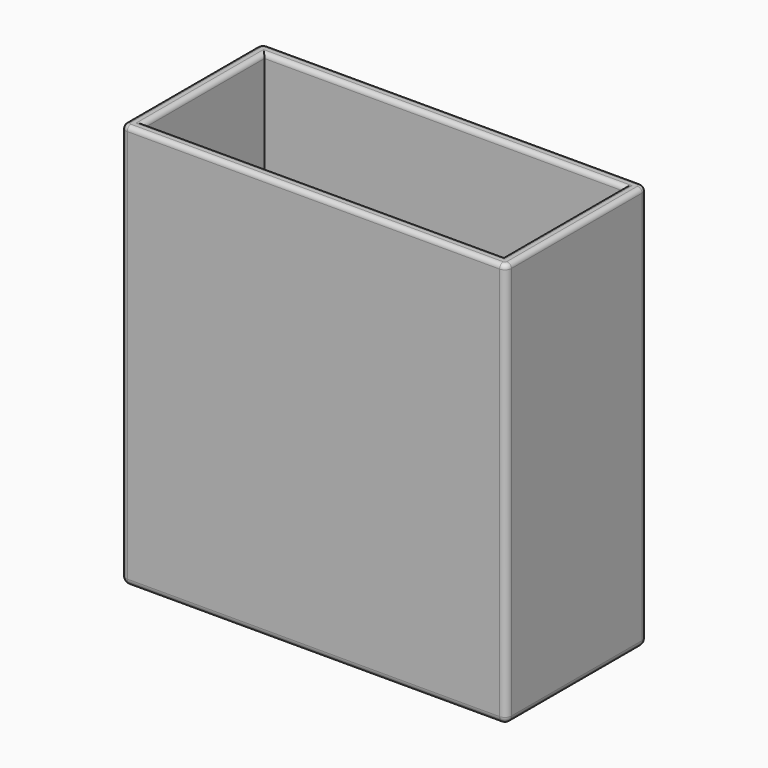
from build123d import *

# Parameters (mm, degrees)
F0_W         = 55
F0_H         = 23
F1_DEPTH     = 60
F2_T         = 2
F3_T1_DEPTH  = 63.5
F3_T3_DEPTH  = 25
F3_T5_DEPTH  = 57
F3_S9_W      = 1
F3_S9_H      = 1
F3_T10_DEPTH = 1
F3_S15_W     = 1
F3_S15_H     = 1
F3_T16_DEPTH = 1
F3_S21_W     = 1
F3_S21_H     = 1
F3_T22_DEPTH = 1
F3_S27_W     = 1
F3_S27_H     = 1
F3_T28_DEPTH = 1
F4_R         = 0.7


# Not quite as in the source:
# - a fillet or chamfer that OpenCascade refuses, or shapes differently, is made with other operations: its cross-section is extruded or revolved along the edge and cut away or added


with BuildPart() as f1:
    # F0 (on Top) → F1 (new body)
    with BuildSketch(Plane.XY):
        Rectangle(F0_W, F0_H)
    extrude(amount=F1_DEPTH)

    # F2
    f2_openings = [f1.faces().sort_by_distance(p)[0] for p in [
        (0, 0, 60),
    ]]
    offset(amount=F2_T, openings=f2_openings, kind=Kind.INTERSECTION)

    # F3: fillet of radius 1 on 8 edges, made by hand

    # F3_s2 → F3_t1 (cut)
    with BuildSketch(Plane.XY.offset(-1)):
        with BuildLine():
            ThreePointArc((29.5, -12.5), (29.2071067812, -13.2071067812), (28.5, -13.5))
            Line((28.5, -13.5), (29.5, -13.5))
            Line((29.5, -13.5), (29.5, -12.5))
        make_face()
        with BuildLine():
            ThreePointArc((29.5, 12.5), (29.2071067812, 13.2071067812), (28.5, 13.5))
            Line((28.5, 13.5), (29.5, 13.5))
            Line((29.5, 13.5), (29.5, 12.5))
        make_face()
        with BuildLine():
            ThreePointArc((-28.5, 13.5), (-29.2071067812, 13.2071067812), (-29.5, 12.5))
            Line((-29.5, 12.5), (-29.5, 13.5))
            Line((-29.5, 13.5), (-28.5, 13.5))
        make_face()
        with BuildLine():
            ThreePointArc((-29.5, -12.5), (-29.2071067812, -13.2071067812), (-28.5, -13.5))
            Line((-28.5, -13.5), (-29.5, -13.5))
            Line((-29.5, -13.5), (-29.5, -12.5))
        make_face()
    extrude(amount=F3_T1_DEPTH, mode=Mode.SUBTRACT)

    # F3_s4 → F3_t3 (cut)
    with BuildSketch(Plane.XZ.offset(-12.5)):
        with BuildLine():
            ThreePointArc((29.5, -1), (29.2071067812, -1.7071067812), (28.5, -2))
            Line((28.5, -2), (29.5, -2))
            Line((29.5, -2), (29.5, -1))
        make_face()
        with BuildLine():
            ThreePointArc((-29.5, -1), (-29.2071067812, -1.7071067812), (-28.5, -2))
            Line((-28.5, -2), (-29.5, -2))
            Line((-29.5, -2), (-29.5, -1))
        make_face()
    extrude(amount=F3_T3_DEPTH, mode=Mode.SUBTRACT)

    # F3_s6 → F3_t5 (cut)
    with BuildSketch(Plane.YZ.offset(-28.5)):
        with BuildLine():
            ThreePointArc((13.5, -1), (13.2071067812, -1.7071067812), (12.5, -2))
            Line((12.5, -2), (13.5, -2))
            Line((13.5, -2), (13.5, -1))
        make_face()
        with BuildLine():
            ThreePointArc((-13.5, -1), (-13.2071067812, -1.7071067812), (-12.5, -2))
            Line((-12.5, -2), (-13.5, -2))
            Line((-13.5, -2), (-13.5, -1))
        make_face()
    extrude(amount=F3_T5_DEPTH, mode=Mode.SUBTRACT)


with BuildPart() as f3_tool8:
    # F3_s9 → F3_t10 (new body)
    with BuildSketch(Plane.XZ.offset(12.5)):
        with Locations((29, -1.5)):
            Rectangle(F3_S9_W, F3_S9_H)
    extrude(amount=F3_T10_DEPTH)

    # F3_s11 → F3_t12 (revolve, cut)
    with BuildSketch(Plane(origin=(28.5, -12.5, -1), x_dir=(-0.7071067812, 0, 0.7071067812), z_dir=(0.7071067812, 0, 0.7071067812))):
        with BuildLine():
            ThreePointArc((0, -1), (1, 0), (0, 1))
            Line((0, 1), (0, -1))
        make_face()
    revolve(axis=Axis((28.5, -12.5, -1), (0, -1, 0)), mode=Mode.SUBTRACT)


with BuildPart() as f1_1:
    add(f1.part)

    # F3_t7: cut F3_tool8
    add(f3_tool8.part, mode=Mode.SUBTRACT)


with BuildPart() as f3_tool14:
    # F3_s15 → F3_t16 (new body)
    with BuildSketch(Plane.XY.offset(-1)):
        with Locations((29, 13)):
            Rectangle(F3_S15_W, F3_S15_H)
    extrude(amount=-F3_T16_DEPTH)

    # F3_s17 → F3_t18 (revolve, cut)
    with BuildSketch(Plane(origin=(28.5, 12.5, -1), x_dir=(-0.7071067812, -0.7071067812, 0), z_dir=(0.7071067812, -0.7071067812, 0))):
        with BuildLine():
            ThreePointArc((0, -1), (1, 0), (0, 1))
            Line((0, 1), (0, -1))
        make_face()
    revolve(axis=Axis((28.5, 12.5, -1), (0, 0, -1)), mode=Mode.SUBTRACT)


with BuildPart() as f1_2:
    add(f1_1.part)

    # F3_t13: cut F3_tool14
    add(f3_tool14.part, mode=Mode.SUBTRACT)


with BuildPart() as f3_tool20:
    # F3_s21 → F3_t22 (new body)
    with BuildSketch(Plane.YZ.offset(-28.5)):
        with Locations((13, -1.5)):
            Rectangle(F3_S21_W, F3_S21_H)
    extrude(amount=-F3_T22_DEPTH)

    # F3_s23 → F3_t24 (revolve, cut)
    with BuildSketch(Plane(origin=(-28.5, 12.5, -1), x_dir=(0, -0.7071067812, 0.7071067812), z_dir=(0, -0.7071067812, -0.7071067812))):
        with BuildLine():
            ThreePointArc((0, -1), (1, 0), (0, 1))
            Line((0, 1), (0, -1))
        make_face()
    revolve(axis=Axis((-28.5, 12.5, -1), (-1, 0, 0)), mode=Mode.SUBTRACT)


with BuildPart() as f1_3:
    add(f1_2.part)

    # F3_t19: cut F3_tool20
    add(f3_tool20.part, mode=Mode.SUBTRACT)


with BuildPart() as f3_tool26:
    # F3_s27 → F3_t28 (new body)
    with BuildSketch(Plane.YZ.offset(-28.5)):
        with Locations((-13, -1.5)):
            Rectangle(F3_S27_W, F3_S27_H)
    extrude(amount=-F3_T28_DEPTH)

    # F3_s29 → F3_t30 (revolve, cut)
    with BuildSketch(Plane(origin=(-28.5, -12.5, -1), x_dir=(0, 0.7071067812, 0.7071067812), z_dir=(0, -0.7071067812, 0.7071067812))):
        with BuildLine():
            ThreePointArc((0, -1), (1, 0), (0, 1))
            Line((0, 1), (0, -1))
        make_face()
    revolve(axis=Axis((-28.5, -12.5, -1), (-1, 0, 0)), mode=Mode.SUBTRACT)


with BuildPart() as f1_4:
    add(f1_3.part)

    # F3_t25: cut F3_tool26
    add(f3_tool26.part, mode=Mode.SUBTRACT)

    # F4
    f4_edges = [f1_4.edges().sort_by_distance(p)[0] for p in [
        (0, -11.5, 60),
        (27.5, 0, 60),
        (0, 11.5, 60),
        (-27.5, 0, 60),
        (0, 13.5, 60),
        (0, -13.5, 60),
        (-29.5, 0, 60),
        (29.5, 0, 60),
        (-29.207107, 13.207107, 60),
        (29.207107, 13.207107, 60),
        (29.207107, -13.207107, 60),
        (-29.207107, -13.207107, 60),
    ]]
    fillet(f4_edges, radius=F4_R)


solid = f1_4.part
